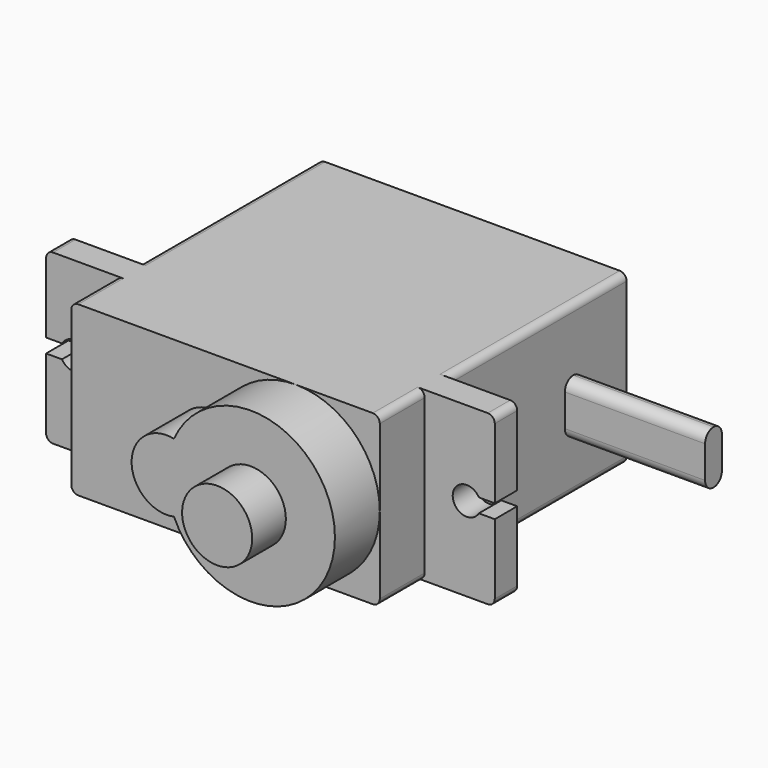
from build123d import *

# Parameters (mm, degrees)
F0_W      = 5
F0_H      = 2
F1_DEPTH  = 12
F2_R      = 0.5
F4_DEPTH  = 4
F5_R      = 2.5
F6_DEPTH  = 3
F7_W      = 1.5
F7_H      = 3.8
F8_DEPTH  = 10
F9_R      = 0.74999
F11_DEPTH = 2


# Not quite as in the source:
# - a fillet or chamfer is up to 0.001 mm smaller than in the source, because OpenCascade refuses the exact size


with BuildPart() as f1:
    # F0 (on Top) → F1 (new body)
    with BuildSketch(Plane.XY):
        Polygon((-11, -11), (11, -11), (11, -7), (11, -5), (11, 11), (-11, 11), (-11, -5), (-11, -7), align=None)
        with Locations((13.5, -6)):
            Rectangle(F0_W, F0_H)
        with Locations((-13.5, -6)):
            Rectangle(F0_W, F0_H)
    extrude(amount=F1_DEPTH)

    # F2
    f2_edges = [f1.edges().sort_by_distance(p)[0] for p in [
        (11, 3, 12),
        (11, -9, 12),
        (-11, -9, 12),
        (16, -6, 12),
        (-11, 3, 12),
        (-16, -6, 12),
        (-11, 3, 0),
        (-11, -9, 0),
        (-16, -6, 0),
        (11, -9, 0),
        (11, 3, 0),
        (16, -6, 0),
    ]]
    fillet(f2_edges, radius=F2_R)

    # F3 (on face) → F4 (join)
    with BuildSketch(Plane.XZ.offset(11)):
        with BuildLine():
            ThreePointArc((-0.4791666667, 3.5548552929), (6.25, 0.1316527028), (11, 6))
            ThreePointArc((11, 6), (6.25, 11.8683472972), (-0.4791666667, 8.4451447071))
            ThreePointArc((-0.4791666667, 8.4451447071), (0.9432039694, 7.572882174), (1.5, 6))
            ThreePointArc((1.5, 6), (0.9432039694, 4.427117826), (-0.4791666667, 3.5548552929))
        make_face()
        with BuildLine():
            ThreePointArc((1.5, 6), (0.9432039694, 7.572882174), (-0.4791666667, 8.4451447071))
            ThreePointArc((-0.4791666667, 8.4451447071), (-1, 6), (-0.4791666667, 3.5548552929))
            ThreePointArc((-0.4791666667, 3.5548552929), (0.9432039694, 4.427117826), (1.5, 6))
        make_face()
        with BuildLine():
            ThreePointArc((-0.4791666667, 3.5548552929), (-1, 6), (-0.4791666667, 8.4451447071))
            ThreePointArc((-0.4791666667, 8.4451447071), (-3.5, 6), (-0.4791666667, 3.5548552929))
        make_face()
    extrude(amount=F4_DEPTH)

    # F10 (on face) → F11 (cut, through all)
    with BuildSketch(Plane.XZ.offset(7)):
        with BuildLine():
            ThreePointArc((14.8660254038, 5.5), (14.9659258263, 5.7411809549), (15, 6))
            ThreePointArc((15, 6), (14.9659258263, 6.2588190451), (14.8660254038, 6.5))
            Line((14.8660254038, 6.5), (14, 6.5))
            Line((14, 6.5), (14, 5.5))
            Line((14, 5.5), (14.8660254038, 5.5))
        make_face()
        with BuildLine():
            Line((14, 6.5), (14.8660254038, 6.5))
            ThreePointArc((14.8660254038, 6.5), (13, 6), (14.8660254038, 5.5))
            Line((14.8660254038, 5.5), (14, 5.5))
            Line((14, 5.5), (14, 6.5))
        make_face()
        with BuildLine():
            ThreePointArc((14.8660254038, 6.5), (14.9659258263, 6.2588190451), (15, 6))
            ThreePointArc((15, 6), (14.9659258263, 5.7411809549), (14.8660254038, 5.5))
            Line((14.8660254038, 5.5), (16, 5.5))
            Line((16, 5.5), (16, 6.5))
            Line((16, 6.5), (14.8660254038, 6.5))
        make_face()
        with BuildLine():
            Line((-14.8660254038, 6.5), (-14, 6.5))
            Line((-14, 6.5), (-14, 5.5))
            Line((-14, 5.5), (-14.8660254038, 5.5))
            ThreePointArc((-14.8660254038, 5.5), (-13.7411809549, 5.0340741737), (-13, 6))
            ThreePointArc((-13, 6), (-13.7411809549, 6.9659258263), (-14.8660254038, 6.5))
        make_face()
        with BuildLine():
            ThreePointArc((-14.8660254038, 5.5), (-15, 6), (-14.8660254038, 6.5))
            Line((-14.8660254038, 6.5), (-16, 6.5))
            Line((-16, 6.5), (-16, 5.5))
            Line((-16, 5.5), (-14.8660254038, 5.5))
        make_face()
        with BuildLine():
            Line((-14, 5.5), (-14, 6.5))
            Line((-14, 6.5), (-14.8660254038, 6.5))
            ThreePointArc((-14.8660254038, 6.5), (-15, 6), (-14.8660254038, 5.5))
            Line((-14.8660254038, 5.5), (-14, 5.5))
        make_face()
    extrude(amount=-F11_DEPTH, mode=Mode.SUBTRACT)


with BuildPart() as f6:
    # F5 (on face) → F6 (new body)
    with BuildSketch(Plane.XZ.offset(15)):
        with Locations((5, 6)):
            Circle(F5_R)
    extrude(amount=F6_DEPTH)


with BuildPart() as f8:
    # F7 (on face) → F8 (new body)
    with BuildSketch(Plane.YZ.offset(11)):
        with Locations((6.25, 5.6300098076)):
            Rectangle(F7_W, F7_H)
    extrude(amount=F8_DEPTH)

    # F9 (radius 0.75 in the source; OpenCascade refuses exactly that, so slightly less here)
    f9_edges = [f8.edges().sort_by_distance(p)[0] for p in [
        (16, 5.5, 7.53001),
        (16, 7, 7.53001),
        (16, 5.5, 3.73001),
        (16, 7, 3.73001),
    ]]
    fillet(f9_edges, radius=F9_R)


solid = Compound([f1.part, f6.part, f8.part])
